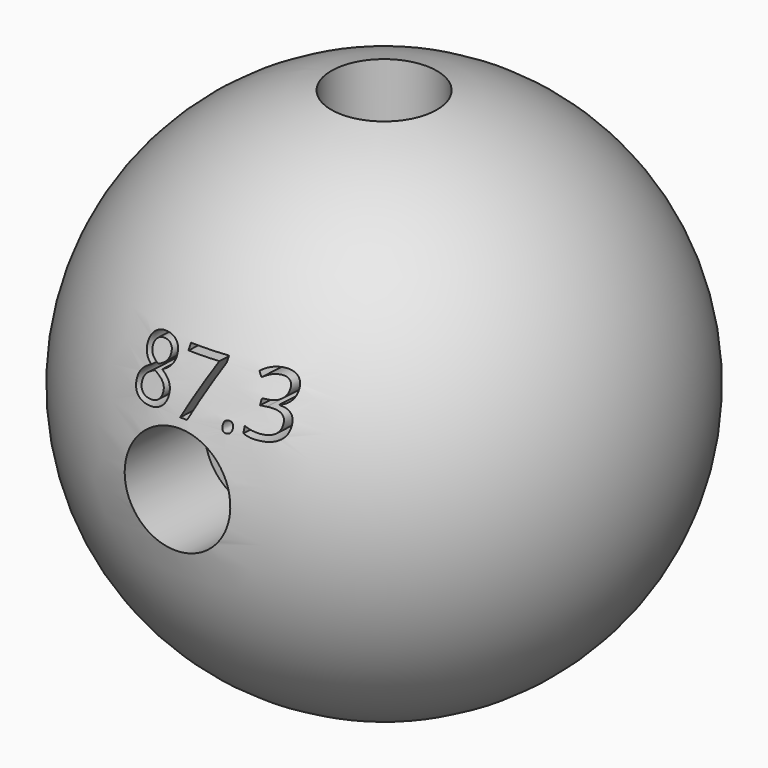
from build123d import *

# Parameters (mm, degrees)
F6_R          = 3.175
F7_DEPTH      = 50.8
F8_ANGLE      = 87.3
F9_ANGLE      = 102.4
F11_ANGLE     = 87.3
F13_TEXT_SIZE = 5.1391705508
F14_DEPTH     = 3.81
F17_TEXT_SIZE = 4.6599688681
F18_DEPTH     = 3.81
F20_TEXT_SIZE = 3.8491070477
F21_DEPTH     = 3.81


# Not quite as in the source:
# - Text() gives the source's letters only with a copy of the font that has no kerning and outlines rounded to 1/6400 em; it was checked with that copy


with BuildPart() as f2:
    # F0 (on Front) → F2 (revolve)
    with BuildSketch(Plane.XZ):
        with BuildLine():
            Line((0, -15.875), (0, 15.875))
            ThreePointArc((0, 15.875), (-15.875, 0), (0, -15.875))
        make_face()
    revolve(axis=Axis((0, 0, 0), (0, 0, 1)))

    # F13 (on offset) → F14 (cut)
    with BuildSketch(Plane(origin=(0, 15.857376765, 0.747814905), x_dir=(-1, 0, 0), z_dir=(0, 0.998889875, 0.0471064507))):
        with Locations((-6.0907113366, 3.9763539098)):
            Text('87.3', F13_TEXT_SIZE, font='Open Sans', text_align=(TextAlign.LEFT, TextAlign.BOTTOM))
    extrude(amount=-F14_DEPTH, mode=Mode.SUBTRACT)

    # F17 (on offset) → F18 (cut)
    with BuildSketch(Plane(origin=(0, -15.857376765, 0.747814905), x_dir=(1, 0, 0), z_dir=(0, -0.998889875, 0.0471064507))):
        with Locations((-3.3861657139, 3.6840173416)):
            Text('87.3', F17_TEXT_SIZE, font='Open Sans', text_align=(TextAlign.LEFT, TextAlign.BOTTOM))
    extrude(amount=-F18_DEPTH, mode=Mode.SUBTRACT)


with BuildPart() as f7:
    # F6 (on offset) → F7 (new body)
    with BuildSketch(Plane.XY.offset(9.525)):
        Circle(F6_R)
    extrude(amount=F7_DEPTH)


with BuildPart() as f8_1:
    # F8: copy of F7
    add(f7.part.rotate(Axis((3.4105647355, 0, 0), (1, 0, 0)), F8_ANGLE))


with BuildPart() as f9_1:
    # F9: copy of F7
    add(f7.part.rotate(Axis((0, -3.1340308487, 0), (0, -1, 0)), F9_ANGLE))


with BuildPart() as f11_1:
    # F11: copy of F7
    add(f7.part.rotate(Axis((-8.2367919385, 0, 0), (-1, 0, 0)), F11_ANGLE))


with BuildPart() as f2_1:
    add(f2.part)

    # F19: cut F7, F8_1, F11_1, F9_1
    add(f7.part, mode=Mode.SUBTRACT)
    add(f8_1.part, mode=Mode.SUBTRACT)
    add(f11_1.part, mode=Mode.SUBTRACT)
    add(f9_1.part, mode=Mode.SUBTRACT)

    # F20 (on offset) → F21 (cut)
    with BuildSketch(Plane(origin=(-15.5046724186, 0, -3.4089233188), x_dir=(0, -1, 0), z_dir=(-0.9766722783, 0, -0.2147353272))):
        with Locations((-5.6106685661, 3.7276358344)):
            Text('102.4', F20_TEXT_SIZE, font='Open Sans', text_align=(TextAlign.LEFT, TextAlign.BOTTOM))
    extrude(amount=-F21_DEPTH, mode=Mode.SUBTRACT)


solid = f2_1.part
